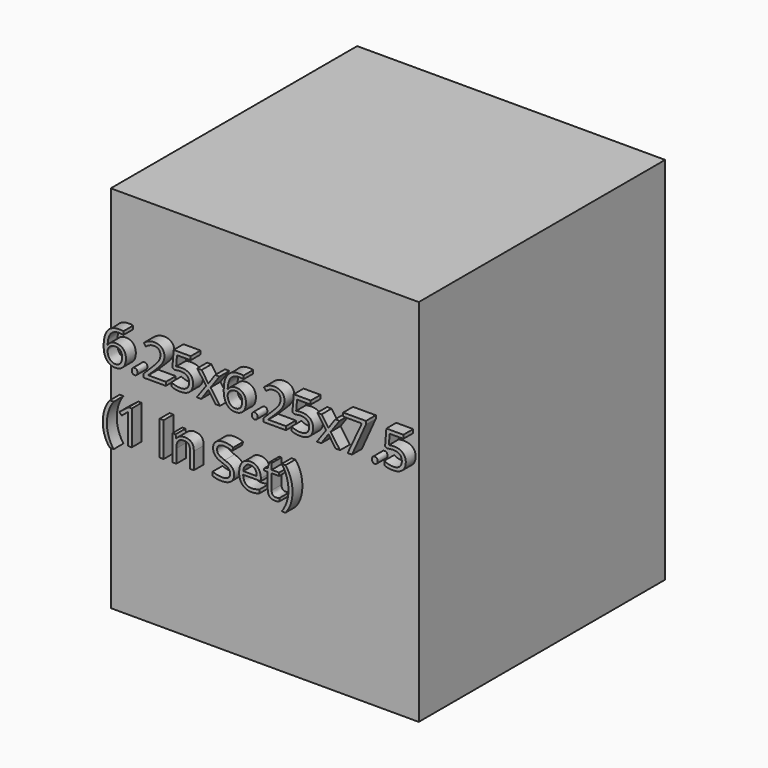
from build123d import *

# Parameters (mm, degrees)
F0_W         = 158.75
F0_H         = 190.5
F1_DEPTH     = 158.75
F2_TEXT_SIZE = 24.6997617543
F3_DEPTH     = 6.35


# Not quite as in the source:
# - Text() gives the source's letters only with a copy of the font that has no kerning and outlines rounded to 1/6400 em; it was checked with that copy


with BuildPart() as f1:
    # F0 (on Front) → F1 (new body)
    with BuildSketch(Plane.XZ):
        with Locations((79.375, 95.25)):
            Rectangle(F0_W, F0_H)
    extrude(amount=F1_DEPTH)

    # F2 (on face) → F3 (join)
    with BuildSketch(Plane.XZ.offset(158.75)):
        with Locations((0, 114.3222623779)):
            Text('6.25x6.25x7.5', F2_TEXT_SIZE, font='Open Sans', text_align=(TextAlign.LEFT, TextAlign.BOTTOM))
        with Locations((0, 80.7305863921)):
            Text('(1 In Set)', F2_TEXT_SIZE, font='Open Sans', text_align=(TextAlign.LEFT, TextAlign.BOTTOM))
    extrude(amount=F3_DEPTH)


solid = f1.part
